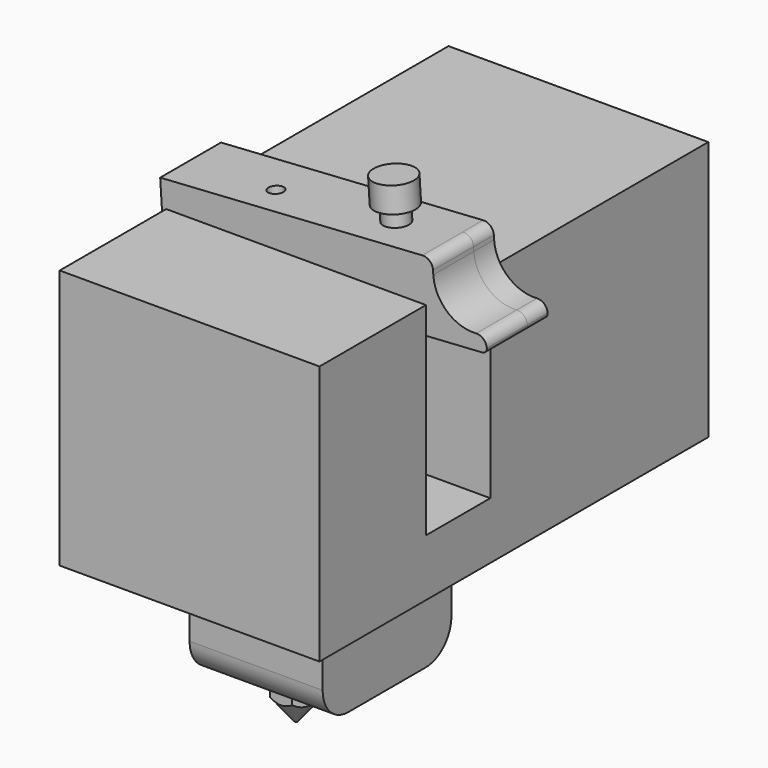
from build123d import *

# Parameters (mm, degrees)
F0_W      = 41
F0_H      = 41
F1_DEPTH  = 43
F2_W      = 41
F2_H      = 9
F3_DEPTH  = 12.7
F5_DEPTH  = 4
F6_R      = 6.35
F7_R      = 1.60019
F8_R      = 1.6002
F9_R      = 0.7874
F11_DEPTH = 8
F12_W     = 41
F12_H     = 41
F13_DEPTH = 21
F15_D     = 2.3876
F15_DEPTH = 12.7
F15_TIP   = 0.717307407
F16_R     = 1.9812
F17_DEPTH = 2.3876
F18_R     = 3.175
F19_DEPTH = 3.9624
F21_DEPTH = 4.7752
F23_R     = 3.175
F24_DEPTH = 21.7254
F28_W     = 21
F28_H     = 25.4
F29_DEPTH = 15.875
F30_R     = 5.08
F32_DEPTH = 6


# Not quite as in the source:
# - a fillet or chamfer is up to 0.001 mm smaller than in the source, because OpenCascade refuses the exact size


with BuildPart() as f1:
    # F0 (on Front) → F1 (new body)
    with BuildSketch(Plane.XZ):
        Rectangle(F0_W, F0_H)
    extrude(amount=F1_DEPTH)

    # F2 (on face) → F3 (join)
    with BuildSketch(Plane.XZ.offset(43)):
        with Locations((0, -16)):
            Rectangle(F2_W, F2_H)
    extrude(amount=F3_DEPTH)

    # F4 (on face) → F5 (join)
    with BuildSketch(Plane.XZ.offset(43)):
        with BuildLine():
            Line((-22.0036495704, 24.0950572902), (-20.4869841684, 0.4436360632))
            ThreePointArc((-20.4869841684, 0.4436360632), (-13.7436360632, -5.4869841684), (-7.8130158316, 1.2563639368))
            Line((-7.8130158316, 1.2563639368), (-8.6257437052, 13.9303322737))
            Line((-8.6257437052, 13.9303322737), (29.5957513579, 16.3813147587))
            Line((29.5957513579, 16.3813147587), (29.4429585176, 18.764020806))
            Line((29.4429585176, 18.764020806), (21.5090543388, 18.2552531571))
            Line((21.5090543388, 18.2552531571), (20.9579096507, 26.85))
            Line((20.9579096507, 26.85), (-22.0036495704, 24.0950572902))
        make_face()
    extrude(amount=F5_DEPTH)

    # F6
    f6_edges = [f1.edges().sort_by_distance(p)[0] for p in [
        (21.509054, -45, 18.255253),
    ]]
    fillet(f6_edges, radius=F6_R)

    # F7 (radius 1.6002 in the source; OpenCascade refuses exactly that, so slightly less here)
    f7_edges = [f1.edges().sort_by_distance(p)[0] for p in [
        (29.442959, -45, 18.764021),
    ]]
    fillet(f7_edges, radius=F7_R)

    # F8
    f8_edges = [f1.edges().sort_by_distance(p)[0] for p in [
        (20.95791, -45, 26.85),
    ]]
    fillet(f8_edges, radius=F8_R)

    # F9
    f9_edges = [f1.edges().sort_by_distance(p)[0] for p in [
        (29.595751, -45, 16.381315),
    ]]
    fillet(f9_edges, radius=F9_R)

    # F10 (on face) → F11 (join)
    with BuildSketch(Plane.XZ.offset(47)):
        with BuildLine():
            Line((19.3609896402, 26.7475962879), (-22.0036495704, 24.0950572902))
            Line((-22.0036495704, 24.0950572902), (-21.2997120421, 13.1176044))
            Line((-21.2997120421, 13.1176044), (-8.6257437052, 13.9303322737))
            Line((-8.6257437052, 13.9303322737), (28.809965321, 16.3309256305))
            ThreePointArc((28.809965321, 16.3309256305), (29.3508413223, 16.5967075264), (29.5453622297, 17.1671007956))
            ThreePointArc((29.5453622297, 17.1671007956), (29.0052248284, 18.2663004111), (27.8460385072, 18.661617094))
            ThreePointArc((27.8460385072, 18.661617094), (23.246092788, 20.2303340893), (21.102690402, 24.5922373256))
            Line((21.102690402, 24.5922373256), (21.0603133628, 25.2530799896))
            ThreePointArc((21.0603133628, 25.2530799896), (20.5201759615, 26.3522796051), (19.3609896402, 26.7475962879))
        make_face()
    extrude(amount=F11_DEPTH)

    # F12 (on face) → F13 (join)
    with BuildSketch(Plane.XZ.offset(55.7)):
        Rectangle(F12_W, F12_H)
    extrude(amount=F13_DEPTH)

    # F15
    with Locations(Plane(origin=(-1.628897193, 0, 25.4016038063), x_dir=(0.9979502627, 0, 0.0639943208), z_dir=(-0.0639943208, 0, 0.9979502627))):
        with Locations((-6.1164010452, -50)):
            Hole(F15_D / 2, depth=F15_DEPTH)
            with Locations((0, 0, -(F15_DEPTH + F15_TIP / 2))):  # 118° drill point
                Cone(0, F15_D / 2, F15_TIP, mode=Mode.SUBTRACT)

    # F16 (on face) → F17 (join)
    with BuildSketch(Plane(origin=(-1.628897193, 0, 25.4016038063), x_dir=(0.9979502627, 0, 0.0639943208), z_dir=(-0.0639943208, 0, 0.9979502627))):
        with Locations((12.1207989548, -49)):
            Circle(F16_R)
    extrude(amount=F17_DEPTH)

    # F18 (on face) → F19 (join)
    with BuildSketch(Plane(origin=(-1.7816900333, 0, 27.7843098536), x_dir=(0.9979502627, 0, 0.0639943208), z_dir=(-0.0639943208, 0, 0.9979502627))):
        with Locations((12.1207989548, -49)):
            Circle(F18_R)
    extrude(amount=F19_DEPTH)

    # F20 (on face) → F21 (join)
    with BuildSketch(Plane(origin=(0, 0, -20.5), x_dir=(1, 0, 0), z_dir=(0, 0, -1))):
        Polygon((-5.7375, 43), (-0.975, 45.749630657), (-0.975, 51.248891971), (-5.7375, 53.9985226281), (-10.5, 51.248891971), (-10.5, 45.749630657), align=None)
    extrude(amount=F21_DEPTH)

    # F23 (on offset) → F24 (join, through all)
    with BuildSketch(Plane(origin=(0, 0, -26.8754), x_dir=(1, 0, 0), z_dir=(0, 0, -1))):
        with Locations((-5.7375, 48.499261314)):
            Circle(F23_R)
    extrude(amount=-F24_DEPTH)

    # F26 (on face) → F27 (revolve)
    with BuildSketch(Plane(origin=(-14.15, 0, 0), x_dir=(0, -1, 0), z_dir=(-1, 0, 0))):
        with BuildLine():
            Line((47.7874, 5.6128158316), (47, 5.6128158316))
            Line((47, 5.6128158316), (47, 0.8630158316))
            Line((47, 0.8630158316), (51.3688, 0.8630158316))
            Line((51.3688, 0.8630158316), (51.3688, 7.2130158316))
            Line((51.3688, 7.2130158316), (50.5814, 7.2130158316))
            ThreePointArc((50.5814, 7.2130158316), (49.5781, 6.392545411), (48.5748, 7.2130158316))
            Line((48.5748, 7.2130158316), (47.7874, 7.2130158316))
            Line((47.7874, 7.2130158316), (47.7874, 5.6128158316))
        make_face()
    revolve(axis=Axis((-14.15, -49.1844, 0.8630158316), (0, -1, 0)))

    # F28 (on face) → F29 (join)
    with BuildSketch(Plane(origin=(0, 0, -26.8754), x_dir=(1, 0, 0), z_dir=(0, 0, -1))):
        with Locations((-5.5, 44)):
            Rectangle(F28_W, F28_H)
    extrude(amount=F29_DEPTH)

    # F30
    f30_edges = [f1.edges().sort_by_distance(p)[0] for p in [
        (-5.5, -56.7, -42.7504),
        (-5.5, -56.7, -26.8754),
        (-5.5, -31.3, -42.7504),
        (-5.5, -31.3, -26.8754),
    ]]
    fillet(f30_edges, radius=F30_R)

    # F31 (on face) → F32 (join)
    with BuildSketch(Plane(origin=(0, 0, -42.7504), x_dir=(1, 0, 0), z_dir=(0, 0, -1))):
        Polygon((-4.0054491924, 45.499261314), (-2.2733983849, 48.499261314), (-4.0054491924, 51.499261314), (-7.4695508076, 51.499261314), (-9.2016016151, 48.499261314), (-7.4695508076, 45.499261314), align=None)
    extrude(amount=F32_DEPTH)

    # F34 (on offset) → F35 (revolve, cut)
    with BuildSketch(Plane.XZ.offset(48.502061314)):
        Polygon((-2.2479983849, -44.7504), (-5.4875, -48.7504), (-2.2479983849, -48.7504), align=None)
    revolve(axis=Axis((-5.7375, -48.502061314, -47.4463791664), (0, 0, 1)), mode=Mode.SUBTRACT)


solid = f1.part
